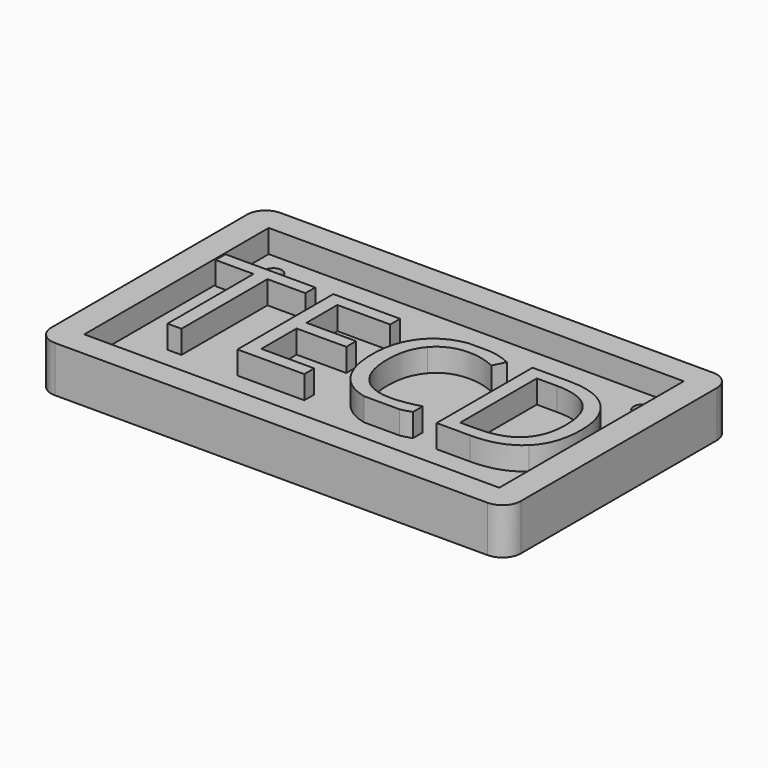
from build123d import *

# Parameters (mm, degrees)
F0_W         = 127
F0_H         = 76.2
F1_DEPTH     = 6.35
F2_R         = 5.08
F4_W         = 129.3370249418
F4_H         = 77.6022149651
F5_DEPTH     = 6.35
F6_R         = 5.08
F7_DEPTH     = 6.35
F8_R         = 2.38125
F9_DEPTH     = 25.4
F10_DEPTH    = 6.35
F11_T1_DEPTH = 31.75


# Not quite as in the source:
# - a fillet or chamfer that OpenCascade refuses, or shapes differently, is made with other operations: its cross-section is extruded or revolved along the edge and cut away or added


with BuildPart() as f1:
    # F0 (on Top) → F1 (new body)
    with BuildSketch(Plane.XY):
        Rectangle(F0_W, F0_H)
    extrude(amount=F1_DEPTH)

    # F2
    f2_edges = [f1.edges().sort_by_distance(p)[0] for p in [
        (-63.5, 38.1, 3.175),
        (-63.5, -38.1, 3.175),
        (63.5, -38.1, 3.175),
        (63.5, 38.1, 3.175),
    ]]
    fillet(f2_edges, radius=F2_R)

    # F4 (on offset) → F5 (join)
    with BuildSketch(Plane.XY.offset(6.35)):
        Rectangle(F4_W, F4_H)
        Polygon((-57.15, -16.6380591357), (-57.15, 16.6380591357), (-57.15, 31.75), (57.15, 31.75), (57.15, 16.6380591357), (57.15, -16.6380591357), (57.15, -31.75), (-57.15, -31.75), align=None, mode=Mode.SUBTRACT)
    extrude(amount=F5_DEPTH)

    # F6
    f6_edges = [f1.edges().sort_by_distance(p)[0] for p in [
        (-64.668512, -38.801107, 9.525),
        (64.668512, 38.801107, 9.525),
        (64.668512, -38.801107, 9.525),
        (-64.668512, 38.801107, 9.525),
    ]]
    fillet(f6_edges, radius=F6_R)

    # F4 (on offset) → F7 (join)
    with BuildSketch(Plane.XY.offset(6.35)):
        Polygon((-46.2962661107, 12.9479340409), (-46.2962661107, -16.6380591357), (-42.4617134193, -16.6380591357), (-42.4617134193, 12.9479340409), (-32.0123768006, 12.9479340409), (-32.0123768006, 16.3564253222), (-56.7456027293, 16.3564253222), (-56.7456027293, 12.9479340409), align=None)
        Polygon((-27.0440674754, 16.3564253222), (-27.0440674754, -16.6380591357), (-8.6512130402, -16.6380591357), (-8.6512130402, -13.2079037149), (-23.2095147839, -13.2079037149), (-23.2095147839, -1.0687642153), (-9.5322213798, -1.0687642153), (-9.5322213798, 2.3180629265), (-23.2095147839, 2.3180629265), (-23.2095147839, 12.9479340409), (-8.6512130402, 12.9479340409), (-8.6512130402, 16.3564253222), align=None)
        with BuildLine():
            Line((15.9701099418, 16.6380591357), (10.0159430302, 16.6380591357))
            add(Edge.make_bspline(
                [(4.3581027293, 14.7496683093), (6.8753977724, 16.2014683592), (10.0159430302, 16.6380591357)],
                knots=[0, 0, 0, 0.6992762354, 0.6992762354, 0.6992762354], degree=2))
            add(Edge.make_bspline(
                [(-1.1481993935, 8.8389689158), (0.7582448825, 12.6735216073), (4.3581027293, 14.7496683093)],
                knots=[0, 0, 0, 1, 1, 1], degree=2))
            add(Edge.make_bspline(
                [(-3.0546436694, -0.0938779378), (-3.0546436694, 5.0044162244), (-1.1481993935, 8.8389689158)],
                knots=[0, 0, 0, 1, 1, 1], degree=2))
            add(Edge.make_bspline(
                [(0.9062831691, -12.6663002274), (-3.0546436694, -8.2395943897), (-3.0546436694, -0.0938779378)],
                knots=[0, 0, 0, 1, 1, 1], degree=2))
            add(Edge.make_bspline(
                [(7.8235797826, -16.6380591357), (3.5974055182, -15.6738809021), (0.9062831691, -12.6663002274)],
                knots=[0.3205826669, 0.3205826669, 0.3205826669, 1, 1, 1], degree=2))
            Line((7.8235797826, -16.6380591357), (17.5614415983, -16.6380591357))
            add(Edge.make_bspline(
                [(20.6170394238, -15.8003790751), (19.2218518782, -16.326144487), (17.5614415983, -16.6380591357)],
                knots=[0, 0, 0, 0.406741787, 0.406741787, 0.406741787], degree=2))
            Line((20.6170394238, -15.8003790751), (20.6170394238, -12.4424374526))
            add(Edge.make_bspline(
                [(12.7385140258, -13.6845147839), (16.1903335861, -13.6845147839), (20.6170394238, -12.4424374526)],
                knots=[0, 0, 0, 1, 1, 1], degree=2))
            add(Edge.make_bspline(
                [(4.0836902957, -10.1496493556), (7.1202805155, -13.6845147839), (12.7385140258, -13.6845147839)],
                knots=[0, 0, 0, 1, 1, 1], degree=2))
            add(Edge.make_bspline(
                [(1.0471000758, -0.1444275967), (1.0471000758, -6.6147839272), (4.0836902957, -10.1496493556)],
                knots=[0, 0, 0, 1, 1, 1], degree=2))
            add(Edge.make_bspline(
                [(4.1956216831, 9.7741376042), (1.0471000758, 6.1526156179), (1.0471000758, -0.1444275967)],
                knots=[0, 0, 0, 1, 1, 1], degree=2))
            add(Edge.make_bspline(
                [(12.7818423048, 13.3956595906), (7.3441432904, 13.3956595906), (4.1956216831, 9.7741376042)],
                knots=[0, 0, 0, 1, 1, 1], degree=2))
            add(Edge.make_bspline(
                [(20.2776345716, 11.6408642911), (16.5297384382, 13.3956595906), (12.7818423048, 13.3956595906)],
                knots=[0, 0, 0, 1, 1, 1], degree=2))
            Line((20.2776345716, 11.6408642911), (21.9024450341, 14.9338134951))
            add(Edge.make_bspline(
                [(15.9701099418, 16.6380591357), (19.2412217115, 16.2297995741), (21.9024450341, 14.9338134951)],
                knots=[0.3150184776, 0.3150184776, 0.3150184776, 1, 1, 1], degree=2))
        make_face()
        with BuildLine():
            Line((27.8167551175, -16.6380591357), (36.9590219864, -16.6380591357))
            add(Edge.make_bspline(
                [(49.7192001516, -12.3160633055), (45.285272934, -16.6380591357), (36.9590219864, -16.6380591357)],
                knots=[0, 0, 0, 1, 1, 1], degree=2))
            add(Edge.make_bspline(
                [(54.1531273692, 0.173313116), (54.1531273692, -7.9940674754), (49.7192001516, -12.3160633055)],
                knots=[0, 0, 0, 1, 1, 1], degree=2))
            add(Edge.make_bspline(
                [(49.8889025777, 12.0922005307), (54.1531273692, 7.8279757392), (54.1531273692, 0.173313116)],
                knots=[0, 0, 0, 1, 1, 1], degree=2))
            add(Edge.make_bspline(
                [(37.926686884, 16.3564253222), (45.6246777862, 16.3564253222), (49.8889025777, 12.0922005307)],
                knots=[0, 0, 0, 1, 1, 1], degree=2))
            Line((37.926686884, 16.3564253222), (27.8167551175, 16.3564253222))
            Line((27.8167551175, 16.3564253222), (27.8167551175, -16.6380591357))
        make_face()
        with BuildLine():
            add(Edge.make_bspline(
                [(50.094711903, 0.0361068992), (50.094711903, 6.4920204701), (46.8559230478, 9.7633055345)],
                knots=[0, 0, 0, 1, 1, 1], degree=2))
            add(Edge.make_bspline(
                [(46.6392816528, -9.9474507202), (50.094711903, -6.5714556482), (50.094711903, 0.0361068992)],
                knots=[0, 0, 0, 1, 1, 1], degree=2))
            add(Edge.make_bspline(
                [(36.323540561, -13.3234457923), (43.1838514026, -13.3234457923), (46.6392816528, -9.9474507202)],
                knots=[0, 0, 0, 1, 1, 1], degree=2))
            Line((36.323540561, -13.3234457923), (31.6513078089, -13.3234457923))
            Line((31.6513078089, -13.3234457923), (31.6513078089, 13.0345905989))
            Line((31.6513078089, 13.0345905989), (37.2262130402, 13.0345905989))
            add(Edge.make_bspline(
                [(46.8559230478, 9.7633055345), (43.6171341926, 13.0345905989), (37.2262130402, 13.0345905989)],
                knots=[0, 0, 0, 1, 1, 1], degree=2))
        make_face(mode=Mode.SUBTRACT)
    extrude(amount=F7_DEPTH)

    # F8 (on face) → F9 (cut)
    with BuildSketch(Plane(origin=(0, 0, 0), x_dir=(1, 0, 0), z_dir=(0, 0, -1))):
        with Locations((-50.8, 25.4)):
            Circle(F8_R)
        with Locations((-50.8, -25.4)):
            Circle(F8_R)
        with Locations((50.8, -25.4)):
            Circle(F8_R)
        with Locations((50.8, 25.4)):
            Circle(F8_R)
    extrude(amount=-F9_DEPTH, mode=Mode.SUBTRACT)

    # F4 (on offset) → F10 (join)
    with BuildSketch(Plane.XY.offset(6.35)):
        Rectangle(F4_W, F4_H)
        Polygon((-57.15, -16.6380591357), (-57.15, 16.6380591357), (-57.15, 31.75), (57.15, 31.75), (57.15, 16.6380591357), (57.15, -16.6380591357), (57.15, -31.75), (-57.15, -31.75), align=None, mode=Mode.SUBTRACT)
    extrude(amount=-F10_DEPTH)

    # F11: fillet of radius 5.08 on 4 edges, made by hand

    # F11_s2 → F11_t1 (cut)
    with BuildSketch(Plane.XY.offset(-12.7)):
        with BuildLine():
            ThreePointArc((-64.6685124709, 33.7211074825), (-63.1806149193, 37.313209931), (-59.5885124709, 38.8011074825))
            Line((-59.5885124709, 38.8011074825), (-64.6685124709, 38.8011074825))
            Line((-64.6685124709, 38.8011074825), (-64.6685124709, 33.7211074825))
        make_face()
        with BuildLine():
            ThreePointArc((-59.5885124709, -38.8011074825), (-63.1806149193, -37.313209931), (-64.6685124709, -33.7211074825))
            Line((-64.6685124709, -33.7211074825), (-64.6685124709, -38.8011074825))
            Line((-64.6685124709, -38.8011074825), (-59.5885124709, -38.8011074825))
        make_face()
        with BuildLine():
            ThreePointArc((59.5885124709, -38.8011074825), (63.1806149193, -37.313209931), (64.6685124709, -33.7211074825))
            Line((64.6685124709, -33.7211074825), (64.6685124709, -38.8011074825))
            Line((64.6685124709, -38.8011074825), (59.5885124709, -38.8011074825))
        make_face()
        with BuildLine():
            ThreePointArc((64.6685124709, 33.7211074825), (63.1806149193, 37.313209931), (59.5885124709, 38.8011074825))
            Line((59.5885124709, 38.8011074825), (64.6685124709, 38.8011074825))
            Line((64.6685124709, 38.8011074825), (64.6685124709, 33.7211074825))
        make_face()
    extrude(amount=F11_T1_DEPTH, mode=Mode.SUBTRACT)


solid = f1.part
